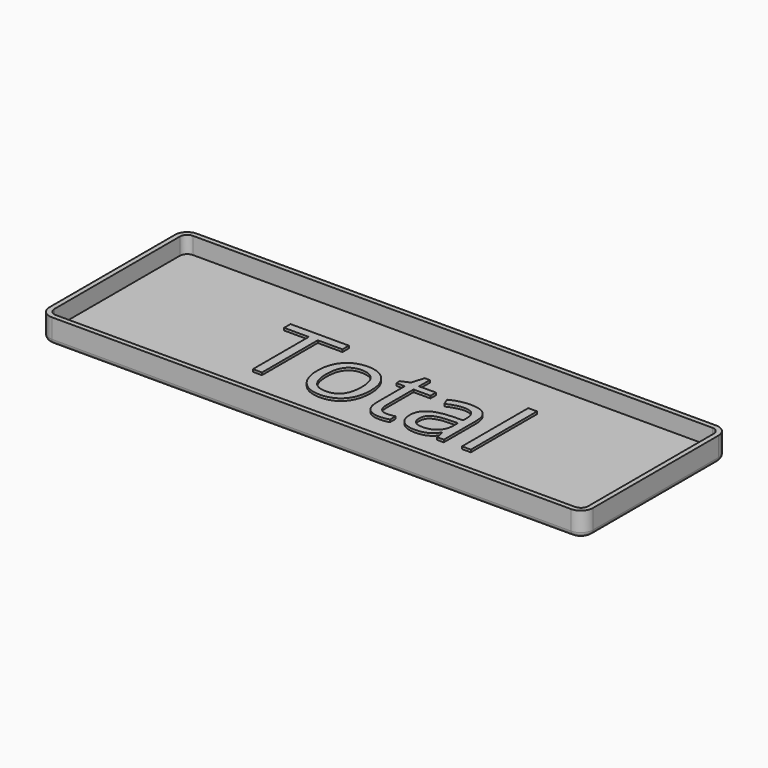
from build123d import *

# Parameters (mm, degrees)
F0_W         = 3.6604817708
F0_H         = 34.2985026042
F1_DEPTH     = 3
F2_DEPTH     = 10
F0_TEXT_SIZE = 45.1388888889
F3_DEPTH     = 4
F4_R         = 2


# Not quite as in the source:
# - Text() gives the source's letters only with a copy of the font that has no kerning and outlines rounded to 1/6400 em; it was checked with that copy


with BuildPart() as f1:
    # F0 (on Top) → F1 (new body)
    with BuildSketch(Plane.XY):
        with BuildLine():
            ThreePointArc((-44.6118305922, 5), (-43.7331509357, 2.8786796564), (-41.6118305922, 2))
            Line((-41.6118305922, 2), (173.3881694078, 2))
            ThreePointArc((173.3881694078, 2), (175.5094897514, 2.8786796564), (176.3881694078, 5))
            Line((176.3881694078, 5), (176.3881694078, 70))
            ThreePointArc((176.3881694078, 70), (175.5094897514, 72.1213203436), (173.3881694078, 73))
            Line((173.3881694078, 73), (-41.6118305922, 73))
            ThreePointArc((-41.6118305922, 73), (-43.7331509357, 72.1213203436), (-44.6118305922, 70))
            Line((-44.6118305922, 70), (-44.6118305922, 5))
        make_face()
        Polygon((28.3629415433, 50.1459418403), (28.3629415433, 21.25), (24.6178243558, 21.25), (24.6178243558, 50.1459418403), (14.412203696, 50.1459418403), (14.412203696, 53.4749348958), (38.568562203, 53.4749348958), (38.568562203, 50.1459418403), align=None, mode=Mode.SUBTRACT)
        with BuildLine():
            add(Edge.make_bspline(
                [(60.7324619426, 42.4758572049), (63.7193868558, 39.1010199653), (63.7193868558, 33.3528645833)],
                knots=[0, 0, 0, 1, 1, 1], degree=2))
            add(Edge.make_bspline(
                [(63.7193868558, 33.3528645833), (63.7193868558, 27.4424913194), (60.7465678453, 24.124077691)],
                knots=[0, 0, 0, 1, 1, 1], degree=2))
            add(Edge.make_bspline(
                [(60.7465678453, 24.124077691), (57.7737488349, 20.8056640625), (52.5263530016, 20.8056640625)],
                knots=[0, 0, 0, 1, 1, 1], degree=2))
            add(Edge.make_bspline(
                [(52.5263530016, 20.8056640625), (49.2819953627, 20.8056640625), (46.7711446683, 22.3291015625)],
                knots=[0, 0, 0, 1, 1, 1], degree=2))
            add(Edge.make_bspline(
                [(46.7711446683, 22.3291015625), (44.2602939738, 23.8525390625), (42.8920214044, 26.6948784722)],
                knots=[0, 0, 0, 1, 1, 1], degree=2))
            add(Edge.make_bspline(
                [(42.8920214044, 26.6948784722), (41.5237488349, 29.5372178819), (41.5237488349, 33.3528645833)],
                knots=[0, 0, 0, 1, 1, 1], degree=2))
            add(Edge.make_bspline(
                [(41.5237488349, 33.3528645833), (41.5237488349, 39.2561848958), (44.4789354669, 42.5534396701)],
                knots=[0, 0, 0, 1, 1, 1], degree=2))
            add(Edge.make_bspline(
                [(44.4789354669, 42.5534396701), (47.4341220988, 45.8506944444), (52.6815179322, 45.8506944444)],
                knots=[0, 0, 0, 1, 1, 1], degree=2))
            add(Edge.make_bspline(
                [(52.6815179322, 45.8506944444), (57.7455370294, 45.8506944444), (60.7324619426, 42.4758572049)],
                knots=[0, 0, 0, 1, 1, 1], degree=2))
        make_face(mode=Mode.SUBTRACT)
        with BuildLine():
            add(Edge.make_bspline(
                [(75.095797446, 24.9986436632), (76.1325813002, 23.8313802083), (77.9381368558, 23.8313802083)],
                knots=[0, 0, 0, 1, 1, 1], degree=2))
            add(Edge.make_bspline(
                [(77.9381368558, 23.8313802083), (78.9114441474, 23.8313802083), (79.8142219252, 23.9724392361)],
                knots=[0, 0, 0, 1, 1, 1], degree=2))
            add(Edge.make_bspline(
                [(79.8142219252, 23.9724392361), (80.716999703, 24.1134982639), (81.2459710572, 24.2686631944)],
                knots=[0, 0, 0, 1, 1, 1], degree=2))
            Line((81.2459710572, 24.2686631944), (81.2459710572, 21.4686414931))
            add(Edge.make_bspline(
                [(81.2459710572, 21.4686414931), (80.6535231405, 21.1865234375), (79.4968391127, 20.99609375)],
                knots=[0, 0, 0, 1, 1, 1], degree=2))
            add(Edge.make_bspline(
                [(79.4968391127, 20.99609375), (78.3401550849, 20.8056640625), (77.4091655016, 20.8056640625)],
                knots=[0, 0, 0, 1, 1, 1], degree=2))
            add(Edge.make_bspline(
                [(77.4091655016, 20.8056640625), (70.4055847724, 20.8056640625), (70.4055847724, 28.1901041667)],
                knots=[0, 0, 0, 1, 1, 1], degree=2))
            Line((70.4055847724, 28.1901041667), (70.4055847724, 42.5640190972))
            Line((70.4055847724, 42.5640190972), (66.9425856405, 42.5640190972))
            Line((66.9425856405, 42.5640190972), (66.9425856405, 44.3272569444))
            Line((66.9425856405, 44.3272569444), (70.4055847724, 45.8506944444))
            Line((70.4055847724, 45.8506944444), (71.9431281752, 51.0064019097))
            Line((71.9431281752, 51.0064019097), (74.0590135919, 51.0064019097))
            Line((74.0590135919, 51.0064019097), (74.0590135919, 45.4063585069))
            Line((74.0590135919, 45.4063585069), (81.0696472724, 45.4063585069))
            Line((81.0696472724, 45.4063585069), (81.0696472724, 42.5640190972))
            Line((81.0696472724, 42.5640190972), (74.0590135919, 42.5640190972))
            Line((74.0590135919, 42.5640190972), (74.0590135919, 28.3452690972))
            add(Edge.make_bspline(
                [(74.0590135919, 28.3452690972), (74.0590135919, 26.1659071181), (75.095797446, 24.9986436632)],
                knots=[0, 0, 0, 1, 1, 1], degree=2))
        make_face(mode=Mode.SUBTRACT)
        with BuildLine():
            Line((103.6390917169, 21.25), (100.9237054322, 21.25))
            Line((100.9237054322, 21.25), (100.1972514391, 24.6918402778))
            Line((100.1972514391, 24.6918402778), (100.0209276544, 24.6918402778))
            add(Edge.make_bspline(
                [(100.0209276544, 24.6918402778), (98.2153720988, 22.4207899306), (96.4203959703, 21.6132269965)],
                knots=[0, 0, 0, 1, 1, 1], degree=2))
            add(Edge.make_bspline(
                [(96.4203959703, 21.6132269965), (94.6254198419, 20.8056640625), (91.9311924113, 20.8056640625)],
                knots=[0, 0, 0, 1, 1, 1], degree=2))
            add(Edge.make_bspline(
                [(91.9311924113, 20.8056640625), (88.3412401544, 20.8056640625), (86.302937203, 22.6605902778)],
                knots=[0, 0, 0, 1, 1, 1], degree=2))
            add(Edge.make_bspline(
                [(86.302937203, 22.6605902778), (84.2646342516, 24.5155164931), (84.2646342516, 27.9291449653)],
                knots=[0, 0, 0, 1, 1, 1], degree=2))
            add(Edge.make_bspline(
                [(84.2646342516, 27.9291449653), (84.2646342516, 35.2430555556), (95.9654806058, 35.595703125)],
                knots=[0, 0, 0, 1, 1, 1], degree=2))
            Line((95.9654806058, 35.595703125), (100.0632453627, 35.7297092014))
            Line((100.0632453627, 35.7297092014), (100.0632453627, 37.2319878472))
            add(Edge.make_bspline(
                [(100.0632453627, 37.2319878472), (100.0632453627, 40.0743272569), (98.8430847724, 41.4284939236)],
                knots=[0, 0, 0, 1, 1, 1], degree=2))
            add(Edge.make_bspline(
                [(98.8430847724, 41.4284939236), (97.6229241822, 42.7826605903), (94.9286967516, 42.7826605903)],
                knots=[0, 0, 0, 1, 1, 1], degree=2))
            add(Edge.make_bspline(
                [(94.9286967516, 42.7826605903), (91.9100335572, 42.7826605903), (88.1014398072, 40.9347873264)],
                knots=[0, 0, 0, 1, 1, 1], degree=2))
            Line((88.1014398072, 40.9347873264), (86.9729675849, 43.7348090278))
            add(Edge.make_bspline(
                [(86.9729675849, 43.7348090278), (88.7573642863, 44.7010633681), (90.8838291301, 45.2511935764)],
                knots=[0, 0, 0, 1, 1, 1], degree=2))
            add(Edge.make_bspline(
                [(90.8838291301, 45.2511935764), (93.0102939738, 45.8013237847), (95.154391196, 45.8013237847)],
                knots=[0, 0, 0, 1, 1, 1], degree=2))
            add(Edge.make_bspline(
                [(95.154391196, 45.8013237847), (99.470797446, 45.8013237847), (101.5549445815, 43.8864474826)],
                knots=[0, 0, 0, 1, 1, 1], degree=2))
            add(Edge.make_bspline(
                [(101.5549445815, 43.8864474826), (103.6390917169, 41.9715711806), (103.6390917169, 37.7398003472)],
                knots=[0, 0, 0, 1, 1, 1], degree=2))
            Line((103.6390917169, 37.7398003472), (103.6390917169, 21.25))
        make_face(mode=Mode.SUBTRACT)
        with Locations((113.0018846856, 38.3992513021)):
            Rectangle(F0_W, F0_H, mode=Mode.SUBTRACT)
    extrude(amount=F1_DEPTH)

    # F0 (on Top) → F2 (join)
    with BuildSketch(Plane.XY):
        with BuildLine():
            Line((173.3881694078, 75), (-41.6118305922, 75))
            ThreePointArc((-41.6118305922, 75), (-45.1473644981, 73.5355339059), (-46.6118305922, 70))
            Line((-46.6118305922, 70), (-46.6118305922, 5))
            ThreePointArc((-46.6118305922, 5), (-45.1473644981, 1.4644660941), (-41.6118305922, 0))
            Line((-41.6118305922, 0), (173.3881694078, 0))
            ThreePointArc((173.3881694078, 0), (176.9237033138, 1.4644660941), (178.3881694078, 5))
            Line((178.3881694078, 5), (178.3881694078, 70))
            ThreePointArc((178.3881694078, 70), (176.9237033138, 73.5355339059), (173.3881694078, 75))
        make_face()
        with BuildLine():
            Line((173.3881694078, 2), (-41.6118305922, 2))
            ThreePointArc((-41.6118305922, 2), (-43.7331509357, 2.8786796564), (-44.6118305922, 5))
            Line((-44.6118305922, 5), (-44.6118305922, 70))
            ThreePointArc((-44.6118305922, 70), (-43.7331509357, 72.1213203436), (-41.6118305922, 73))
            Line((-41.6118305922, 73), (173.3881694078, 73))
            ThreePointArc((173.3881694078, 73), (175.5094897514, 72.1213203436), (176.3881694078, 70))
            Line((176.3881694078, 70), (176.3881694078, 5))
            ThreePointArc((176.3881694078, 5), (175.5094897514, 2.8786796564), (173.3881694078, 2))
        make_face(mode=Mode.SUBTRACT)
    extrude(amount=F2_DEPTH)



with BuildPart() as f1b:
    # F0 (on Top) → F1, piece 2 (new body)
    with BuildSketch(Plane.XY):
        with BuildLine():
            add(Edge.make_bspline(
                [(89.3004415433, 24.8646375868), (90.4994432794, 23.8313802083), (92.6576464044, 23.8313802083)],
                knots=[0, 0, 0, 1, 1, 1], degree=2))
            add(Edge.make_bspline(
                [(92.6576464044, 23.8313802083), (96.078327828, 23.8313802083), (98.028468887, 25.7039388021)],
                knots=[0, 0, 0, 1, 1, 1], degree=2))
            add(Edge.make_bspline(
                [(98.028468887, 25.7039388021), (99.978609946, 27.5764973958), (99.978609946, 30.9478081597)],
                knots=[0, 0, 0, 1, 1, 1], degree=2))
            Line((99.978609946, 30.9478081597), (99.978609946, 33.1271701389))
            Line((99.978609946, 33.1271701389), (96.3181281752, 32.9790581597))
            add(Edge.make_bspline(
                [(96.3181281752, 32.9790581597), (91.9523512655, 32.8238932292), (90.0268955363, 31.6213650174)],
                knots=[0, 0, 0, 1, 1, 1], degree=2))
            add(Edge.make_bspline(
                [(90.0268955363, 31.6213650174), (88.1014398072, 30.4188368056), (88.1014398072, 27.8868272569)],
                knots=[0, 0, 0, 1, 1, 1], degree=2))
            add(Edge.make_bspline(
                [(88.1014398072, 27.8868272569), (88.1014398072, 25.8978949653), (89.3004415433, 24.8646375868)],
                knots=[0, 0, 0, 1, 1, 1], degree=2))
        make_face()
    extrude(amount=F1_DEPTH)


with BuildPart() as f1c:
    # F0 (on Top) → F1, piece 3 (new body)
    with BuildSketch(Plane.XY):
        with BuildLine():
            add(Edge.make_bspline(
                [(47.1484775676, 40.3811306424), (45.3182366822, 38.0219184028), (45.3182366822, 33.3528645833)],
                knots=[0, 0, 0, 1, 1, 1], degree=2))
            add(Edge.make_bspline(
                [(45.3182366822, 33.3528645833), (45.3182366822, 28.7190755208), (47.1696364217, 26.2963867187)],
                knots=[0, 0, 0, 1, 1, 1], degree=2))
            add(Edge.make_bspline(
                [(47.1696364217, 26.2963867187), (49.0210361613, 23.8736979167), (52.6109884183, 23.8736979167)],
                knots=[0, 0, 0, 1, 1, 1], degree=2))
            add(Edge.make_bspline(
                [(52.6109884183, 23.8736979167), (56.2079936266, 23.8736979167), (58.0699727933, 26.2858072917)],
                knots=[0, 0, 0, 1, 1, 1], degree=2))
            add(Edge.make_bspline(
                [(58.0699727933, 26.2858072917), (59.9319519599, 28.6979166667), (59.9319519599, 33.3528645833)],
                knots=[0, 0, 0, 1, 1, 1], degree=2))
            add(Edge.make_bspline(
                [(59.9319519599, 33.3528645833), (59.9319519599, 37.9584418403), (58.0699727933, 40.3493923611)],
                knots=[0, 0, 0, 1, 1, 1], degree=2))
            add(Edge.make_bspline(
                [(58.0699727933, 40.3493923611), (56.2079936266, 42.7403428819), (52.5686707099, 42.7403428819)],
                knots=[0, 0, 0, 1, 1, 1], degree=2))
            add(Edge.make_bspline(
                [(52.5686707099, 42.7403428819), (48.978718453, 42.7403428819), (47.1484775676, 40.3811306424)],
                knots=[0, 0, 0, 1, 1, 1], degree=2))
        make_face()
    extrude(amount=F1_DEPTH)


with BuildPart() as f1_1:
    add(f1.part)

    add(f1b.part)  # F3 merges F1b

    add(f1c.part)  # F3 merges F1c
    # F0 (on Top) → F3 (join)
    with BuildSketch(Plane.XY):
        with Locations((14.0172384183, 21.25)):
            Text('Total', F0_TEXT_SIZE, font='Open Sans', text_align=(TextAlign.LEFT, TextAlign.BOTTOM))
    extrude(amount=F3_DEPTH)

    # F4
    f4_edges = [f1_1.edges().sort_by_distance(p)[0] for p in [
        (65.888169, 75, 0),
    ]]
    fillet(f4_edges, radius=F4_R)


solid = f1_1.part
